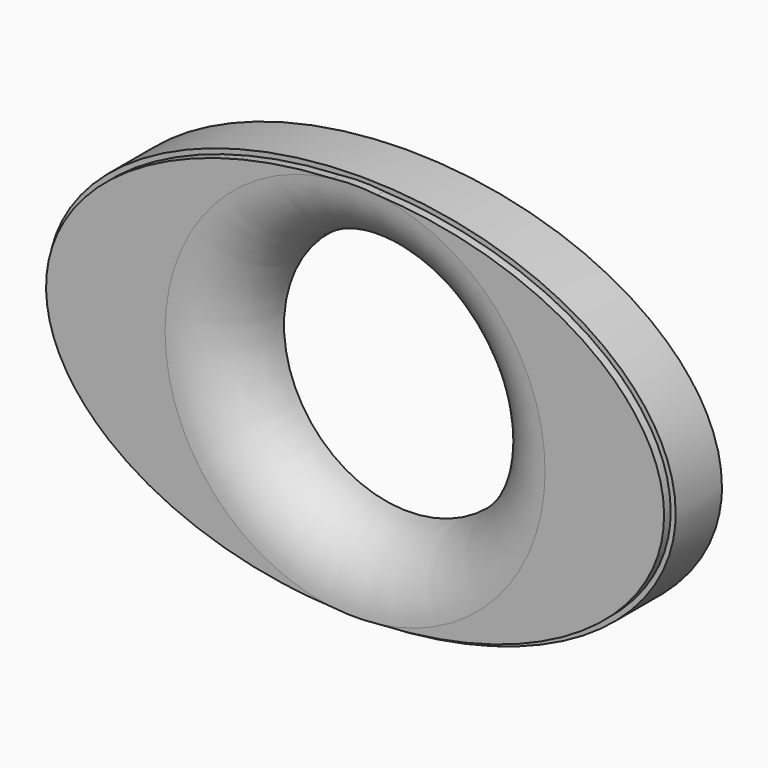
from build123d import *

# Parameters (mm, degrees)
F0_R     = 15
F1_DEPTH = 8
F2_R     = 7.99999
F4_DEPTH = 1


# Not quite as in the source:
# - a fillet or chamfer is up to 0.001 mm smaller than in the source, because OpenCascade refuses the exact size
# - the dataset's text gives a spline's control points without its knots; the knots are read off the source's solid


with BuildPart() as f1:
    # F0 (on Front) → F1 (new body)
    with BuildSketch(Plane.XZ):
        with BuildLine():
            add(Edge.make_bspline(
                [(38, 0), (38, 40.7031939779), (-19, 20.3515969889), (-76, 0), (-19, -20.3515969889), (38, -40.7031939779), (38, 0)],
                knots=[0, 0, 0, 2.0943951024, 2.0943951024, 4.1887902048, 4.1887902048, 6.2831853072, 6.2831853072, 6.2831853072], degree=2, weights=[1, 0.5, 1, 0.5, 1, 0.5, 1]))
        make_face()
        Circle(F0_R, mode=Mode.SUBTRACT)
    extrude(amount=-F1_DEPTH)

    # F2 (radius 8 in the source; OpenCascade refuses exactly that, so slightly less here)
    f2_edges = [f1.edges().sort_by_distance(p)[0] for p in [
        (-15, 0, 0),
    ]]
    fillet(f2_edges, radius=F2_R)

    # F3 (on face) → F4 (cut)
    with BuildSketch(Plane.XZ):
        with BuildLine():
            add(Edge.make_bspline(
                [(38, 0), (38, 40.7031939779), (-19, 20.3515969889), (-76, 0), (-19, -20.3515969889), (38, -40.7031939779), (38, 0)],
                knots=[0, 0, 0, 2.0943951024, 2.0943951024, 4.1887902048, 4.1887902048, 6.2831853072, 6.2831853072, 6.2831853072], degree=2, weights=[1, 0.5, 1, 0.5, 1, 0.5, 1]))
        make_face()
        with BuildLine():
            add(Edge.make_bspline(
                [(37.4, 0), (37.4, 0.3729058543), (37.3700150225, 1.1187175629), (37.1916659495, 2.5989137585), (36.7494239841, 4.429002048), (35.8750924916, 6.5796899728), (34.6638131377, 8.6715326302), (33.1226752034, 10.6890391548), (31.2597201987, 12.6157908188), (29.4459901124, 14.1320344278), (27.8437614939, 15.2824930058), (26.5655992555, 16.1132749708), (25.2206981065, 16.9046504688), (23.3539925194, 17.898962984), (20.885344135, 19.0285928454), (17.7332695204, 20.1944866576), (14.4163055348, 21.1638203846), (10.9598159017, 21.9295641088), (7.38924551, 22.4849605857), (4.6172060854, 22.7412747637), (3.0484899282, 22.8245022324), (2.7121032493, 22.8395279278)],
                knots=[0, 0, 0, 0, 0.0078125, 0.015625, 0.03125, 0.046875, 0.0625, 0.078125, 0.09375, 0.109375, 0.1171875, 0.125, 0.1328125, 0.140625, 0.15625, 0.171875, 0.1875, 0.203125, 0.21875, 0.234375, 0.2386279027, 0.2386279027, 0.2386279027, 0.2386279027], degree=3))
            add(Edge.make_bspline(
                [(2.7121032493, -22.8395279278), (3.0484899282, -22.8245022324), (4.6172060854, -22.7412747637), (7.38924551, -22.4849605857), (10.9598159017, -21.9295641088), (14.4163055348, -21.1638203846), (17.7332695204, -20.1944866576), (20.885344135, -19.0285928454), (23.3539925194, -17.898962984), (25.2206981065, -16.9046504688), (26.5655992555, -16.1132749708), (27.8437614939, -15.2824930058), (29.4459901124, -14.1320344278), (31.2597201987, -12.6157908188), (33.1226752034, -10.6890391548), (34.6638131377, -8.6715326302), (35.8750924916, -6.5796899728), (36.7494239841, -4.429002048), (37.1916659495, -2.5989137585), (37.3700150225, -1.1187175629), (37.4, -0.3729058543), (37.4, 0)],
                knots=[0.7613720973, 0.7613720973, 0.7613720973, 0.7613720973, 0.765625, 0.78125, 0.796875, 0.8125, 0.828125, 0.84375, 0.859375, 0.8671875, 0.875, 0.8828125, 0.890625, 0.90625, 0.921875, 0.9375, 0.953125, 0.96875, 0.984375, 0.9921875, 1, 1, 1, 1], degree=3))
            ThreePointArc((2.7121032493, -22.8395279278), (0, -22.99999), (-2.7121032493, -22.8395279278))
            add(Edge.make_bspline(
                [(-2.7121032493, 22.8395279278), (-3.0484899282, 22.8245022324), (-4.6172060854, 22.7412747637), (-7.38924551, 22.4849605857), (-10.9598159017, 21.9295641088), (-14.4163055348, 21.1638203846), (-17.7332695204, 20.1944866576), (-20.885344135, 19.0285928454), (-23.3539925194, 17.898962984), (-25.2206981065, 16.9046504688), (-26.5655992555, 16.1132749708), (-27.8437614939, 15.2824930058), (-29.4459901124, 14.1320344278), (-31.2597201987, 12.6157908188), (-33.1226752034, 10.6890391548), (-34.6638131377, 8.6715326302), (-35.8750924916, 6.5796899728), (-36.7494239841, 4.429002048), (-37.1916659495, 2.5989137585), (-37.3700150225, 1.1187175629), (-37.4149924887, 0), (-37.3700150225, -1.1187175629), (-37.1916659495, -2.5989137585), (-36.7494239841, -4.429002048), (-35.8750924916, -6.5796899728), (-34.6638131377, -8.6715326302), (-33.1226752034, -10.6890391548), (-31.2597201987, -12.6157908188), (-29.4459901124, -14.1320344278), (-27.8437614939, -15.2824930058), (-26.5655992555, -16.1132749708), (-25.2206981065, -16.9046504688), (-23.3539925194, -17.898962984), (-20.885344135, -19.0285928454), (-17.7332695204, -20.1944866576), (-14.4163055348, -21.1638203846), (-10.9598159017, -21.9295641088), (-7.38924551, -22.4849605857), (-4.6172060854, -22.7412747637), (-3.0484899282, -22.8245022324), (-2.7121032493, -22.8395279278)],
                knots=[0.2613720973, 0.2613720973, 0.2613720973, 0.2613720973, 0.265625, 0.28125, 0.296875, 0.3125, 0.328125, 0.34375, 0.359375, 0.3671875, 0.375, 0.3828125, 0.390625, 0.40625, 0.421875, 0.4375, 0.453125, 0.46875, 0.484375, 0.4921875, 0.5, 0.5078125, 0.515625, 0.53125, 0.546875, 0.5625, 0.578125, 0.59375, 0.609375, 0.6171875, 0.625, 0.6328125, 0.640625, 0.65625, 0.671875, 0.6875, 0.703125, 0.71875, 0.734375, 0.7386279027, 0.7386279027, 0.7386279027, 0.7386279027], degree=3))
            ThreePointArc((-2.7121032493, 22.8395279278), (0, 22.99999), (2.7121032493, 22.8395279278))
        make_face(mode=Mode.SUBTRACT)
    extrude(amount=-F4_DEPTH, mode=Mode.SUBTRACT)


solid = f1.part
